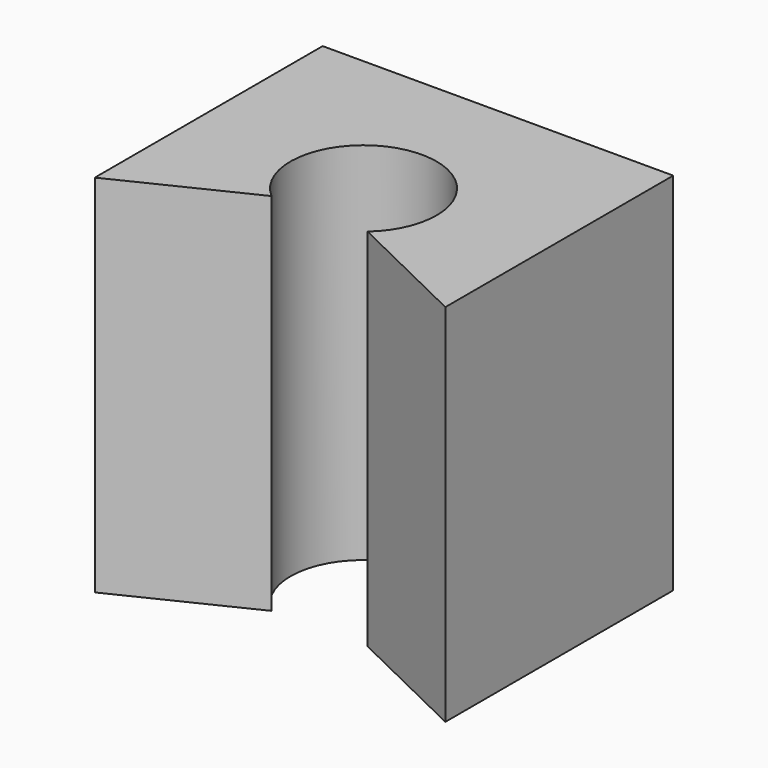
from build123d import *

# Parameters (mm, degrees)
F1_DEPTH = 50
F3_D     = 6.6
F3_DEPTH = 20
F3_TIP   = 1.9828400428


# Not quite as in the source:
# - a feature names something its author has since deleted; it is built from what else it names


with BuildPart() as f1:
    # F0 (on Top) → F1 (new body)
    with BuildSketch(Plane.XY):
        with BuildLine():
            Line((0, 39), (0, 0))
            Line((0, 0), (17.4234656395, 8.4667937898))
            ThreePointArc((17.4234656395, 8.4667937898), (24, 26), (30.5765343605, 8.4667937898))
            Line((30.5765343605, 8.4667937898), (48, 0))
            Line((48, 0), (48, 39))
            Line((48, 39), (0, 39))
        make_face()
    extrude(amount=F1_DEPTH)

    # F3
    with Locations(Plane(origin=(0, 39, 0), x_dir=(-1, 0, 0), z_dir=(0, 1, 0))):
        with Locations((-41.5, 42.5), (-41.5, 7.5), (-6.5, 7.5), (-6.5, 42.5)):
            Hole(F3_D / 2, depth=F3_DEPTH)
            with Locations((0, 0, -(F3_DEPTH + F3_TIP / 2))):  # 118° drill point
                Cone(0, F3_D / 2, F3_TIP, mode=Mode.SUBTRACT)


solid = f1.part
